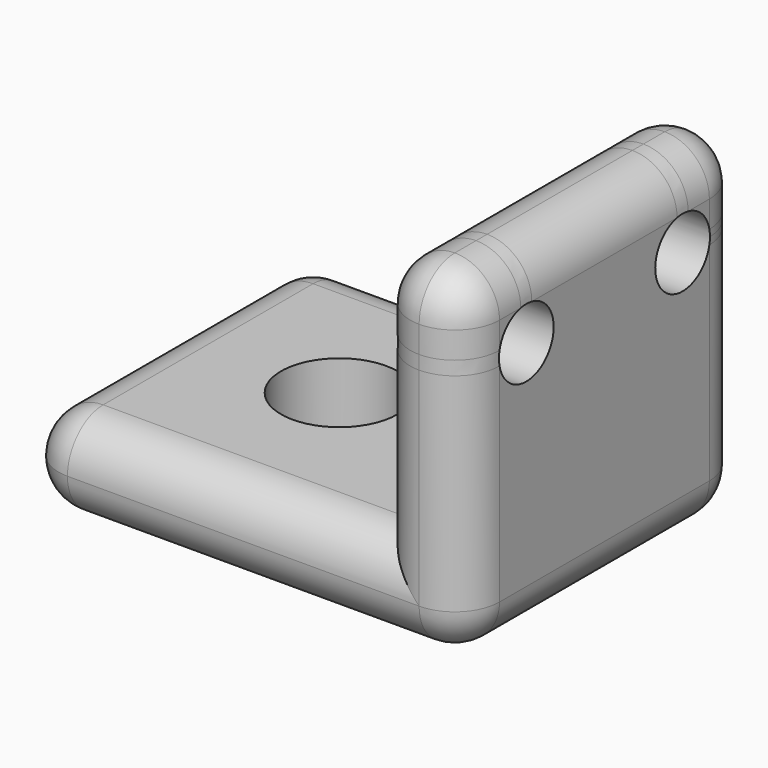
from build123d import *

# Parameters (mm, degrees)
F0_W     = 18
F0_H     = 4.572
F1_DEPTH = 18
F2_R     = 2.9845
F3_DEPTH = 25.4
F4_R     = 1.75
F5_DEPTH = 25.4
F6_R     = 2.28599


# Not quite as in the source:
# - a fillet or chamfer is up to 0.001 mm smaller than in the source, because OpenCascade refuses the exact size


with BuildPart() as f1:
    # F0 (on Front) → F1 (new body)
    with BuildSketch(Plane.XZ):
        Polygon((5.9780351967, 9.1414450236), (5.9780351967, -3.5585549764), (5.9780351967, -8.1305549764), (10.5500351967, -8.1305549764), (10.5500351967, 9.1414450236), align=None)
        with Locations((-3.0219648033, -5.8445549764)):
            Rectangle(F0_W, F0_H)
    extrude(amount=F1_DEPTH)

    # F2 (on face) → F3 (cut)
    with BuildSketch(Plane.XY.offset(-3.5585549764)):
        with Locations((-3.0219648033, -9)):
            Circle(F2_R)
    extrude(amount=-F3_DEPTH, mode=Mode.SUBTRACT)

    # F4 (on face) → F5 (cut)
    with BuildSketch(Plane.YZ.offset(10.5500351967)):
        with Locations((-14, 5.1414450236)):
            Circle(F4_R)
        with Locations((-4, 5.1414450236)):
            Circle(F4_R)
    extrude(amount=-F5_DEPTH, mode=Mode.SUBTRACT)

    # F6 (radius 2.286 in the source; OpenCascade refuses exactly that, so slightly less here)
    f6_edges = [f1.edges().sort_by_distance(p)[0] for p in [
        (8.264035, -18, 9.141445),
        (8.264035, 0, 9.141445),
        (-12.021965, -18, -5.844555),
        (-12.021965, 0, -5.844555),
        (5.978035, -18, 2.791445),
        (-3.021965, -18, -3.558555),
        (-0.735965, -18, -8.130555),
        (10.550035, -18, 0.505445),
        (5.978035, 0, 2.791445),
        (-3.021965, 0, -3.558555),
        (-0.735965, 0, -8.130555),
        (10.550035, 0, 0.505445),
        (-12.021965, -9, -3.558555),
        (-12.021965, -9, -8.130555),
        (10.550035, -9, -8.130555),
        (10.550035, -9, 9.141445),
        (5.978035, -9, 9.141445),
    ]]
    fillet(f6_edges, radius=F6_R)


solid = f1.part
